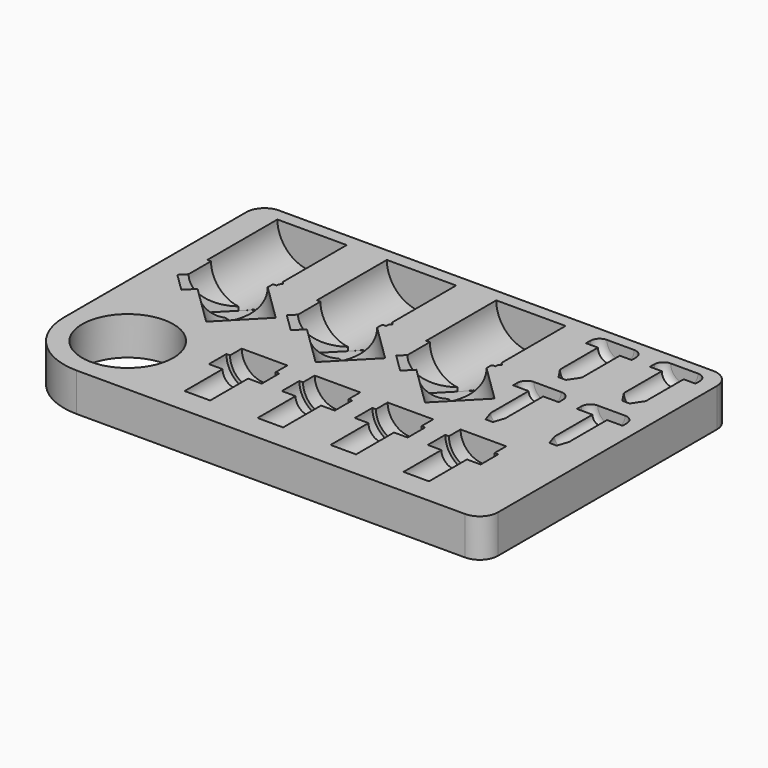
from build123d import *

# Parameters (mm, degrees)
F0_R          = 12.5
F1_DEPTH      = 10.5
F10_START     = -9.5
F9_R          = 12.5
F10_DEPTH     = 1
F19_TEXT_SIZE = 5.5555555556
F20_DEPTH     = 1
F21_R         = 12.5
F22_DEPTH     = 5


# Not quite as in the source:
# - Text() gives the source's letters only with a copy of the font that has no kerning and outlines rounded to 1/6400 em; it was checked with that copy


with BuildPart() as f1:
    # F0 (on Top) → F1 (new body)
    with BuildSketch(Plane.XY):
        with BuildLine():
            ThreePointArc((0, 17.5), (5.1256313292, 5.1256313292), (17.5, 0))
            Line((17.5, 0), (124, 0))
            ThreePointArc((124, 0), (127.5355339059, 1.4644660941), (129, 5))
            Line((129, 5), (129, 80))
            ThreePointArc((129, 80), (127.5355339059, 83.5355339059), (124, 85))
            Line((124, 85), (5, 85))
            ThreePointArc((5, 85), (1.4644660941, 83.5355339059), (0, 80))
            Line((0, 80), (0, 17.5))
        make_face()
        with Locations((17.5, 17.5)):
            Circle(F0_R, mode=Mode.SUBTRACT)
    extrude(amount=F1_DEPTH)

    # F2 (on face) → F3 (revolve, cut)
    with BuildSketch(Plane.XY.offset(10.5)):
        Polygon((14.3187418757, 55.9630800428), (16.818928037, 53.5137803146), (16.818928037, 81.5137803146), (7.318928037, 81.5137803146), (7.318928037, 57.5137803146), (8.318928037, 57.5137803146), (8.318928037, 53.1566108629), (8.318928037, 49.8386146061), align=None)
        Polygon((8.318928037, 49.5137803146), (16.818928037, 53.5137803146), (14.3187418757, 55.9630800428), (8.318928037, 49.8386146061), align=None)
    revolve(axis=Axis((16.818928037, 67.5137803146, 10.5), (0, 1, 0)), mode=Mode.SUBTRACT)

    # F2 (on face) → F4 (revolve, cut)
    with BuildSketch(Plane.XY.offset(10.5)):
        Polygon((44.3187418757, 55.9630800428), (46.818928037, 53.5137803146), (46.818928037, 81.5137803146), (37.318928037, 81.5137803146), (37.318928037, 57.5137803146), (38.318928037, 57.5137803146), (38.318928037, 49.8386146061), align=None)
    revolve(axis=Axis((46.818928037, 67.5137803146, 10.5), (0, 1, 0)), mode=Mode.SUBTRACT)

    # F2 (on face) → F5 (revolve, cut)
    with BuildSketch(Plane.XY.offset(10.5)):
        Polygon((74.3187418757, 55.9630800428), (76.818928037, 53.5137803146), (76.818928037, 81.5137803146), (67.318928037, 81.5137803146), (67.318928037, 57.5137803146), (68.318928037, 57.5137803146), (68.318928037, 49.8386146061), align=None)
    revolve(axis=Axis((76.818928037, 67.5137803146, 10.5), (0, 1, 0)), mode=Mode.SUBTRACT)

    # F2 (on face) → F6 (revolve, cut)
    with BuildSketch(Plane.XY.offset(10.5)):
        Polygon((14.0706147806, 45.7069388121), (25, 35), (30.2484994177, 40.3575417742), (16.818928037, 53.5137803146), (8.318928037, 49.5137803146), (8.318928037, 49.8386146061), (6.6209427297, 48.1053521073), (11.6213150523, 43.2067526508), align=None)
        Polygon((8.318928037, 49.5137803146), (16.818928037, 53.5137803146), (14.3187418757, 55.9630800428), (8.318928037, 49.8386146061), align=None)
    revolve(axis=Axis((22.2836206467, 48.1603109085, 10.5), (0.7143389032, -0.6997999224, 0)), mode=Mode.SUBTRACT)

    # F2 (on face) → F7 (revolve, cut)
    with BuildSketch(Plane.XY.offset(10.5)):
        Polygon((60.2484994177, 40.3575417742), (46.818928037, 53.5137803146), (38.318928037, 49.5137803146), (38.318928037, 49.8386146061), (36.6209427297, 48.1053521073), (41.6213150523, 43.2067526508), (44.0706147806, 45.7069388121), (55, 35), align=None)
        Polygon((38.318928037, 49.5137803146), (46.818928037, 53.5137803146), (44.3187418757, 55.9630800428), (38.318928037, 49.8386146061), align=None)
    revolve(axis=Axis((53.5337137273, 46.9356610444, 10.5), (0.7143389032, -0.6997999224, 0)), mode=Mode.SUBTRACT)

    # F2 (on face) → F8 (revolve, cut)
    with BuildSketch(Plane.XY.offset(10.5)):
        Polygon((90.2484994177, 40.3575417742), (76.818928037, 53.5137803146), (68.318928037, 49.5137803146), (68.318928037, 49.8386146061), (66.6209427297, 48.1053521073), (71.6213150523, 43.2067526508), (74.0706147806, 45.7069388121), (85, 35), align=None)
        Polygon((68.318928037, 49.5137803146), (76.818928037, 53.5137803146), (74.3187418757, 55.9630800428), (68.318928037, 49.8386146061), align=None)
    revolve(axis=Axis((83.5337137273, 46.9356610444, 10.5), (0.7143389032, -0.6997999224, 0)), mode=Mode.SUBTRACT)

    # F9 (on face) → F10 (join)
    with BuildSketch(Plane.XY.offset(10.5).offset(F10_START)):
        with BuildLine():
            ThreePointArc((129, 80), (127.5355339059, 83.5355339059), (124, 85))
            Line((124, 85), (5, 85))
            ThreePointArc((5, 85), (1.4644660941, 83.5355339059), (0, 80))
            Line((0, 80), (0, 17.5))
            ThreePointArc((0, 17.5), (5.1256313292, 5.1256313292), (17.5, 0))
            Line((17.5, 0), (124, 0))
            ThreePointArc((124, 0), (127.5355339059, 1.4644660941), (129, 5))
            Line((129, 5), (129, 80))
        make_face()
        with Locations((17.5, 17.5)):
            Circle(F9_R, mode=Mode.SUBTRACT)
    extrude(amount=-F10_DEPTH)

    # F11 (on face) → F12 (revolve, cut)
    with BuildSketch(Plane.XY.offset(10.5)):
        with BuildLine():
            Line((104.75, 82), (101, 82))
            Line((101, 82), (101, 78))
            Line((101, 78), (101, 72))
            Line((101, 72), (101, 62))
            Line((101, 62), (102, 62))
            Line((102, 62), (104, 65))
            Line((104, 65), (104, 78))
            Line((104, 78), (107.25, 78))
            Line((107.25, 78), (107.25, 79.5))
            ThreePointArc((107.25, 79.5), (106.517766953, 81.267766953), (104.75, 82))
        make_face()
        with BuildLine():
            Line((104.75, 57), (101, 57))
            Line((101, 57), (101, 53))
            Line((101, 53), (101, 37))
            Line((101, 37), (102, 37))
            Line((102, 37), (103, 40))
            Line((103, 40), (103, 53))
            Line((103, 53), (107.25, 53))
            Line((107.25, 53), (107.25, 54.5))
            ThreePointArc((107.25, 54.5), (106.517766953, 56.267766953), (104.75, 57))
        make_face()
    revolve(axis=Axis((101, 45, 10.5), (0, -1, 0)), mode=Mode.SUBTRACT)

    # F11 (on face) → F13 (revolve, cut)
    with BuildSketch(Plane.XY.offset(10.5)):
        Polygon((121.5, 78), (118.5, 78), (118.5, 62), (119.5, 62), (121.5, 65), align=None)
        with BuildLine():
            Line((122.25, 82), (118.5, 82))
            Line((118.5, 82), (118.5, 78))
            Line((118.5, 78), (121.5, 78))
            Line((121.5, 78), (124.75, 78))
            Line((124.75, 78), (124.75, 79.5))
            ThreePointArc((124.75, 79.5), (124.017766953, 81.267766953), (122.25, 82))
        make_face()
        with BuildLine():
            Line((122.25, 57), (118.5, 57))
            Line((118.5, 57), (118.5, 53))
            Line((118.5, 53), (118.5, 37))
            Line((118.5, 37), (119.5, 37))
            Line((119.5, 37), (120.5, 40))
            Line((120.5, 40), (120.5, 53))
            Line((120.5, 53), (124.75, 53))
            Line((124.75, 53), (124.75, 54.5))
            ThreePointArc((124.75, 54.5), (124.017766953, 56.267766953), (122.25, 57))
        make_face()
    revolve(axis=Axis((118.5, 45, 10.5), (0, -1, 0)), mode=Mode.SUBTRACT)

    # F14 (on face) → F15 (revolve, cut)
    with BuildSketch(Plane.XY.offset(10.5)):
        Polygon((51.25, 30), (45, 30), (45, 26), (45, 20), (45, 17.5), (45, 7), (48.5, 7), (48.5, 20), (52.25, 20), (52.25, 26), (51.25, 26), align=None)
    revolve(axis=Axis((45, 13.5, 10.5), (0, -1, 0)), mode=Mode.SUBTRACT)

    # F14 (on face) → F16 (revolve, cut)
    with BuildSketch(Plane.XY.offset(10.5)):
        Polygon((71.25, 30), (65, 30), (65, 26), (65, 20), (65, 7), (68.5, 7), (68.5, 20), (72.25, 20), (72.25, 26), (71.25, 26), align=None)
    revolve(axis=Axis((65, 13.5, 10.5), (0, -1, 0)), mode=Mode.SUBTRACT)

    # F14 (on face) → F17 (revolve, cut)
    with BuildSketch(Plane.XY.offset(10.5)):
        Polygon((91.25, 30), (85, 30), (85, 26), (85, 20), (85, 7), (88.5, 7), (88.5, 20), (92.25, 20), (92.25, 26), (91.25, 26), align=None)
    revolve(axis=Axis((85, 13.5, 10.5), (0, -1, 0)), mode=Mode.SUBTRACT)

    # F14 (on face) → F18 (revolve, cut)
    with BuildSketch(Plane.XY.offset(10.5)):
        Polygon((111.25, 30), (105, 30), (105, 26), (105, 20), (105, 7), (108.5, 7), (108.5, 20), (112.25, 20), (112.25, 26), (111.25, 26), align=None)
    revolve(axis=Axis((105, 13.5, 10.5), (0, -1, 0)), mode=Mode.SUBTRACT)

    # F19 (on face) → F20 (cut)
    with BuildSketch(Plane(origin=(0, 0, 0), x_dir=(1, 0, 0), z_dir=(0, 0, -1))):
        with Locations((30, -9)):
            Text('974, 975', F19_TEXT_SIZE, font='Open Sans', text_align=(TextAlign.LEFT, TextAlign.BOTTOM))
    extrude(amount=-F20_DEPTH, mode=Mode.SUBTRACT)

    # F21 (on face) → F22 (join)
    with BuildSketch(Plane.XY.offset(10.5)):
        with BuildLine():
            Line((0, 80), (0, 17.5))
            ThreePointArc((0, 17.5), (5.1256313292, 5.1256313292), (17.5, 0))
            Line((17.5, 0), (124, 0))
            ThreePointArc((124, 0), (127.5355339059, 1.4644660941), (129, 5))
            Line((129, 5), (129, 80))
            ThreePointArc((129, 80), (127.5355339059, 83.5355339059), (124, 85))
            Line((124, 85), (5, 85))
            ThreePointArc((5, 85), (1.4644660941, 83.5355339059), (0, 80))
        make_face()
        with Locations((17.5, 17.5)):
            Circle(F21_R, mode=Mode.SUBTRACT)
        Polygon((52.25, 26), (52.25, 20), (48.5, 20), (48.5, 7), (41.5, 7), (41.5, 20), (37.75, 20), (37.75, 26), (38.75, 26), (38.75, 30), (51.25, 30), (51.25, 26), align=None, mode=Mode.SUBTRACT)
        Polygon((57.75, 26), (58.75, 26), (58.75, 30), (71.25, 30), (71.25, 26), (72.25, 26), (72.25, 20), (68.5, 20), (68.5, 7), (61.5, 7), (61.5, 20), (57.75, 20), align=None, mode=Mode.SUBTRACT)
        Polygon((88.5, 7), (81.5, 7), (81.5, 20), (77.75, 20), (77.75, 26), (78.75, 26), (78.75, 30), (91.25, 30), (91.25, 26), (92.25, 26), (92.25, 20), (88.5, 20), align=None, mode=Mode.SUBTRACT)
        Polygon((98.75, 26), (98.75, 30), (111.25, 30), (111.25, 26), (112.25, 26), (112.25, 20), (108.5, 20), (108.5, 7), (101.5, 7), (101.5, 20), (97.75, 20), (97.75, 26), align=None, mode=Mode.SUBTRACT)
        Polygon((25.318928037, 55.6859994852), (35.4969988354, 45.7150835485), (25, 35), (14.0706147806, 45.7069388121), (11.6213150523, 43.2067526508), (6.6209427297, 48.1053521073), (8.318928037, 49.8386146061), (8.318928037, 57.5137803146), (7.318928037, 57.5137803146), (7.318928037, 81.5137803146), (26.318928037, 81.5137803146), (26.318928037, 59.6059876939), (27.0169133442, 58.9222085218), (26.318928037, 58.209721934), (26.318928037, 57.5137803146), (25.6371509574, 57.5137803146), (25.318928037, 57.188946023), align=None, mode=Mode.SUBTRACT)
        Polygon((37.318928037, 81.5137803146), (56.318928037, 81.5137803146), (56.318928037, 59.6059876939), (57.0169133442, 58.9222085218), (56.318928037, 58.209721934), (56.318928037, 57.5137803146), (55.6371509574, 57.5137803146), (55.318928037, 57.188946023), (55.318928037, 55.6859994852), (65.4969988354, 45.7150835485), (55, 35), (44.0706147806, 45.7069388121), (41.6213150523, 43.2067526508), (36.6209427297, 48.1053521073), (38.318928037, 49.8386146061), (38.318928037, 57.5137803146), (37.318928037, 57.5137803146), align=None, mode=Mode.SUBTRACT)
        Polygon((85.318928037, 55.6859994852), (95.4969988354, 45.7150835485), (85, 35), (74.0706147806, 45.7069388121), (71.6213150523, 43.2067526508), (66.6209427297, 48.1053521073), (68.318928037, 49.8386146061), (68.318928037, 57.5137803146), (67.318928037, 57.5137803146), (67.318928037, 81.5137803146), (86.318928037, 81.5137803146), (86.318928037, 59.6059876939), (87.0169133442, 58.9222085218), (86.318928037, 58.209721934), (86.318928037, 57.5137803146), (85.6371509574, 57.5137803146), (85.318928037, 57.188946023), align=None, mode=Mode.SUBTRACT)
        with BuildLine():
            Line((107.25, 53), (103, 53))
            Line((103, 53), (103, 40))
            Line((103, 40), (102, 37))
            Line((102, 37), (100, 37))
            Line((100, 37), (99, 40))
            Line((99, 40), (99, 53))
            Line((99, 53), (94.75, 53))
            Line((94.75, 53), (94.75, 54.5))
            ThreePointArc((94.75, 54.5), (95.482233047, 56.267766953), (97.25, 57))
            Line((97.25, 57), (104.75, 57))
            ThreePointArc((104.75, 57), (106.517766953, 56.267766953), (107.25, 54.5))
            Line((107.25, 54.5), (107.25, 53))
        make_face(mode=Mode.SUBTRACT)
        with BuildLine():
            Line((124.75, 53), (120.5, 53))
            Line((120.5, 53), (120.5, 40))
            Line((120.5, 40), (119.5, 37))
            Line((119.5, 37), (117.5, 37))
            Line((117.5, 37), (116.5, 40))
            Line((116.5, 40), (116.5, 53))
            Line((116.5, 53), (112.25, 53))
            Line((112.25, 53), (112.25, 54.5))
            ThreePointArc((112.25, 54.5), (112.982233047, 56.267766953), (114.75, 57))
            Line((114.75, 57), (122.25, 57))
            ThreePointArc((122.25, 57), (124.017766953, 56.267766953), (124.75, 54.5))
            Line((124.75, 54.5), (124.75, 53))
        make_face(mode=Mode.SUBTRACT)
        with BuildLine():
            Line((107.25, 78), (104, 78))
            Line((104, 78), (104, 65))
            Line((104, 65), (102, 62))
            Line((102, 62), (100, 62))
            Line((100, 62), (98, 65))
            Line((98, 65), (98, 78))
            Line((98, 78), (94.75, 78))
            Line((94.75, 78), (94.75, 79.5))
            ThreePointArc((94.75, 79.5), (95.482233047, 81.267766953), (97.25, 82))
            Line((97.25, 82), (104.75, 82))
            ThreePointArc((104.75, 82), (106.517766953, 81.267766953), (107.25, 79.5))
            Line((107.25, 79.5), (107.25, 78))
        make_face(mode=Mode.SUBTRACT)
        with BuildLine():
            Line((119.5, 62), (117.5, 62))
            Line((117.5, 62), (115.5, 65))
            Line((115.5, 65), (115.5, 78))
            Line((115.5, 78), (112.25, 78))
            Line((112.25, 78), (112.25, 79.5))
            ThreePointArc((112.25, 79.5), (112.982233047, 81.267766953), (114.75, 82))
            Line((114.75, 82), (122.25, 82))
            ThreePointArc((122.25, 82), (124.017766953, 81.267766953), (124.75, 79.5))
            Line((124.75, 79.5), (124.75, 78))
            Line((124.75, 78), (121.5, 78))
            Line((121.5, 78), (121.5, 65))
            Line((121.5, 65), (119.5, 62))
        make_face(mode=Mode.SUBTRACT)
    extrude(amount=-F22_DEPTH)


solid = f1.part
